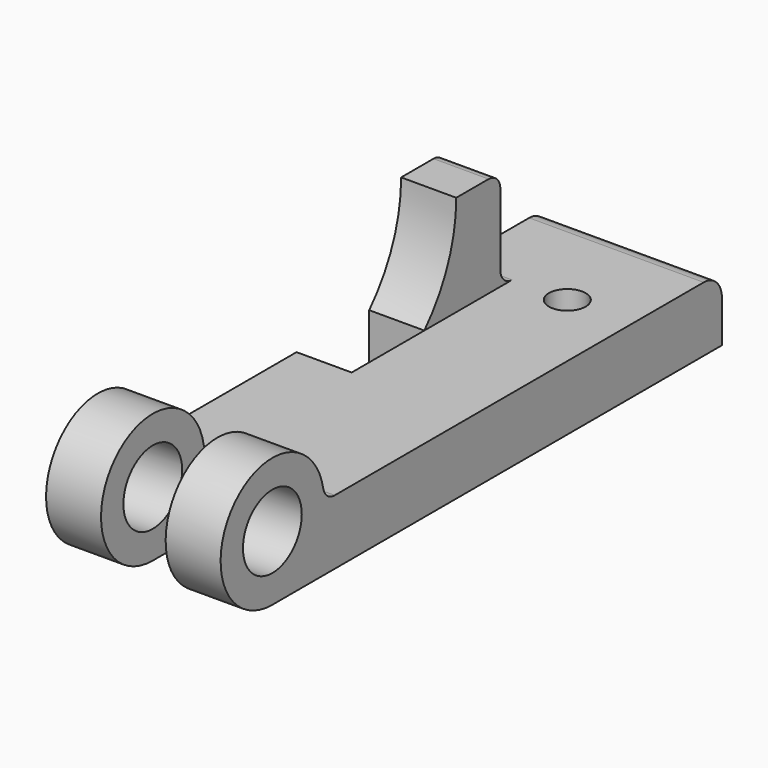
from build123d import *

# Parameters (mm, degrees)
F0_R      = 12.7
F1_DEPTH  = 60.325
F2_DEPTH  = 41.275
F0_W      = 32.8422
F0_H      = 22.352
F4_DEPTH  = 41.275
F5_DEPTH  = 19.05
F0_W_2    = 44.1198
F6_DEPTH  = 41.275
F7_DEPTH  = 19.05
F8_W      = 22.3266
F8_H      = 44.704
F9_DEPTH  = 47.752
F10_R     = 6.35
F11_DEPTH = 22.352
F12_R     = 5.08
F13_R     = 7.874
F14_W     = 22.2758
F14_H     = 4.605526296
F15_DEPTH = 22.352


with BuildPart() as f1:
    # F0 (on Right) → F1 (new body)
    with BuildSketch(Plane.YZ):
        with BuildLine():
            ThreePointArc((-94.8944, 22.352), (-133.0516507731, 38.1572507731), (-117.2464, 0))
            Line((-117.2464, 0), (-25.4, 0))
            Line((-25.4, 0), (-31.3944, 22.352))
            Line((-31.3944, 22.352), (-94.8944, 22.352))
        make_face()
        with Locations((-117.2464, 22.352)):
            Circle(F0_R, mode=Mode.SUBTRACT)
    extrude(amount=-F1_DEPTH)

    # F0 (on Right) → F2 (join)
    with BuildSketch(Plane.YZ):
        Polygon((-31.3944, 22.352), (-25.4, 0), (0, 0), (0, 22.352), align=None)
    extrude(amount=-F2_DEPTH)


with BuildPart() as f1_1:
    # F3: moved
    add(f1.part.moved(Location((41.275, 0, 0))))

    # F0 (on Right) → F4 (join)
    with BuildSketch(Plane.YZ):
        with Locations((16.4211, 11.176)):
            Rectangle(F0_W, F0_H)
    extrude(amount=F4_DEPTH)

    # F0 (on Right) → F5 (join)
    with BuildSketch(Plane.YZ):
        with Locations((16.4211, 11.176)):
            Rectangle(F0_W, F0_H)
        with BuildLine():
            ThreePointArc((13.7922, 57.15), (10.2180153616, 38.4343576341), (0, 22.352))
            Line((0, 22.352), (32.8422, 22.352))
            Line((32.8422, 22.352), (32.8422, 57.15))
            Line((32.8422, 57.15), (13.7922, 57.15))
        make_face()
    extrude(amount=-F5_DEPTH)

    # F0 (on Right) → F6 (join)
    with BuildSketch(Plane.YZ):
        with Locations((54.9021, 11.176)):
            Rectangle(F0_W_2, F0_H)
    extrude(amount=F6_DEPTH)

    # F0 (on Right) → F7 (join)
    with BuildSketch(Plane.YZ):
        with Locations((54.9021, 11.176)):
            Rectangle(F0_W_2, F0_H)
    extrude(amount=-F7_DEPTH)

    # F8 (on Top) → F9 (cut)
    with BuildSketch(Plane.XY):
        with Locations((11.1125, -117.2464)):
            Rectangle(F8_W, F8_H)
    extrude(amount=F9_DEPTH, mode=Mode.SUBTRACT)

    # F10 (on face) → F11 (cut)
    with BuildSketch(Plane.XY.offset(22.352)):
        with Locations((18.923, 38.1)):
            Circle(F10_R)
    extrude(amount=-F11_DEPTH, mode=Mode.SUBTRACT)

    # F12
    f12_edges = [f1_1.edges().sort_by_distance(p)[0] for p in [
        (-9.525, 32.8422, 57.15),
        (-9.525, 32.8422, 22.352),
        (-9.5504, -94.8944, 22.352),
        (31.7754, -94.8944, 22.352),
    ]]
    fillet(f12_edges, radius=F12_R)

    # F13
    f13_edges = [f1_1.edges().sort_by_distance(p)[0] for p in [
        (11.1125, 76.962, 22.352),
    ]]
    fillet(f13_edges, radius=F13_R)

    # F14 (on face) → F15 (cut)
    with BuildSketch(Plane.XY.offset(22.352)):
        with Locations((11.1379, -92.591636852)):
            Rectangle(F14_W, F14_H)
    extrude(amount=-F15_DEPTH, mode=Mode.SUBTRACT)


solid = f1_1.part
